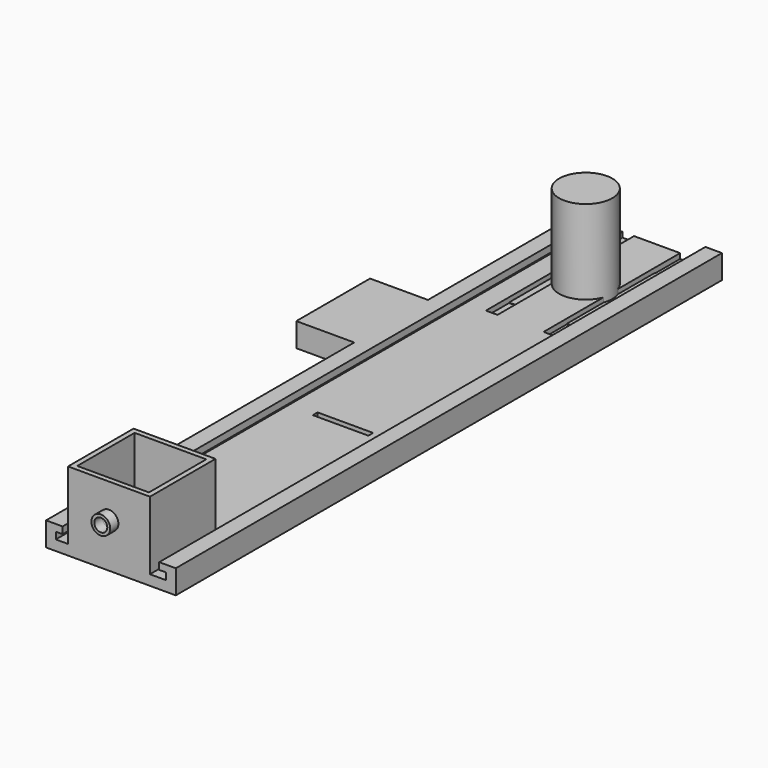
from build123d import *

# Parameters (mm, degrees)
F0_W           = 32.25
F0_H           = 32.23
F1_DEPTH       = 1.65
F2_R           = 7.8
F3_DEPTH       = 26
F4_W           = 38
F4_H           = 200
F5_DEPTH       = 3
F7_DEPTH       = 200
F8_W           = 24
F8_H           = 24
F8_W_2         = 21
F8_H_2         = 21
F9_DEPTH       = 20
F10_W          = 17
F10_H          = 27
F11_DEPTH      = 4
F11_DEPTH_BACK = 3
F12_W          = 16.2802226841
F12_H          = 1.756504178
F13_DEPTH      = 3
F14_W          = 3.4
F14_H          = 50
F15_DEPTH      = 1.5
F16_DEPTH      = 3
F17_R          = 2.75
F17_R_2        = 1.9
F18_DEPTH      = 3
F19_DEPTH      = 1.5


with BuildPart() as f1:
    # F0 (on Top) → F1 (new body)
    with BuildSketch(Plane.XY):
        Rectangle(F0_W, F0_H)
    extrude(amount=F1_DEPTH)

    # F2 (on face) → F3 (join)
    with BuildSketch(Plane.XY.offset(1.65)):
        Circle(F2_R)
    extrude(amount=F3_DEPTH)


with BuildPart() as f5:
    # F4 (on Top) → F5 (new body)
    with BuildSketch(Plane.XY):
        with Locations((0.5689565417, -74.5901823044)):
            Rectangle(F4_W, F4_H)
    extrude(amount=F5_DEPTH)

    # F6 (on face) → F7 (join, through all)
    with BuildSketch(Plane(origin=(0, 25.4098176956, 0), x_dir=(-1, 0, 0), z_dir=(0, 1, 0))):
        Polygon((-19.5689565417, 3), (-16.7189565417, 3), (-16.7189565417, 5), (-14.7189565417, 5), (-14.7189565417, 7), (-19.5689565417, 7), align=None)
        Polygon((15.5810434583, 5), (15.5810434583, 3), (18.4310434583, 3), (18.4310434583, 7), (13.5810434583, 7), (13.5810434583, 5), align=None)
    extrude(amount=-F7_DEPTH)

    # F8 (on face) → F9 (join)
    with BuildSketch(Plane.XY.offset(3)):
        with Locations((0, -162.5901823044)):
            Rectangle(F8_W, F8_H)
        with Locations((0, -162.5901823044)):
            Rectangle(F8_W_2, F8_H_2, mode=Mode.SUBTRACT)
    extrude(amount=F9_DEPTH)

    # F10 (on face) → F11 (join, two sides)
    with BuildSketch(Plane.XY.offset(3)) as f11_sk:
        with Locations((-26.9029508382, -48.2411993444)):
            Rectangle(F10_W, F10_H)
    extrude(amount=F11_DEPTH)
    extrude(f11_sk.sketch, amount=-F11_DEPTH_BACK)

    # F12 (on face) → F13 (cut, through all)
    with BuildSketch(Plane(origin=(0, 0, 0), x_dir=(1, 0, 0), z_dir=(0, 0, -1))):
        with Locations((0, 88.90273422)):
            Rectangle(F12_W, F12_H)
    extrude(amount=-F13_DEPTH, mode=Mode.SUBTRACT)

    # F14 (on face) → F15 (cut)
    with BuildSketch(Plane.XY.offset(3)):
        with Locations((-7.8810434583, 0.4098176956)):
            Rectangle(F14_W, F14_H)
        with Locations((9.0189565417, 0.4098176956)):
            Rectangle(F14_W, F14_H)
    extrude(amount=-F15_DEPTH, mode=Mode.SUBTRACT)

    # F16 (cut, through all): a face of the model
    f16_faces = [f5.faces().sort_by_distance(p)[0] for p in [
        (0, -162.5901823044, 3),
    ]]
    extrude(f16_faces, amount=-F16_DEPTH, mode=Mode.SUBTRACT)

    # F17 (on face) → F18 (join)
    with BuildSketch(Plane.XZ.offset(174.5901823044)):
        with Locations((0, 13)):
            Circle(F17_R)
        with Locations((0, 13)):
            Circle(F17_R_2, mode=Mode.SUBTRACT)
    extrude(amount=F18_DEPTH)

    # F19 (cut, through all): a face of the model
    f19_faces = [f5.faces().sort_by_distance(p)[0] for p in [
        (0, -174.5901823044, 13),
    ]]
    extrude(f19_faces, amount=-F19_DEPTH, mode=Mode.SUBTRACT)


solid = Compound([f1.part, f5.part])
